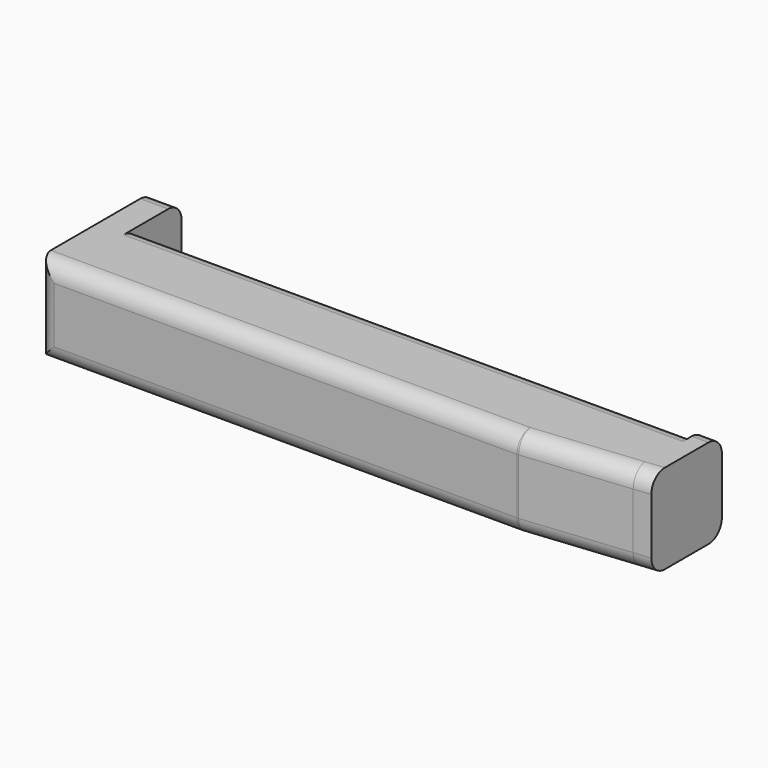
from build123d import *

# Parameters (mm, degrees)
F2_DEPTH      = 8
F2_DEPTH_BACK = 8
F3_R          = 3


# Not quite as in the source:
# - two fillets or chamfers of one size are made in one step


with BuildPart() as f2:
    # F1 (on Top) → F2 (new body, two sides)
    with BuildSketch(Plane.XY) as f2_sk:
        Polygon((-55, -8), (-50, -8), (-50, 8), (-50, 18), (-55, 18), align=None)
        Polygon((-50, -8), (30.9022613208, -8), (50, -6.0806050441), (50, 8), (-50, 8), align=None)
        Polygon((50, 8), (50, -6.0806050441), (53, -5.7790936996), (53, 10), (50, 10), align=None)
    extrude(amount=F2_DEPTH)
    extrude(f2_sk.sketch, amount=-F2_DEPTH_BACK)

    # F3 (call 1 of 7: OpenCascade refuses the feature's edges together)
    f3_edges = [f2.edges().sort_by_distance(p)[0] for p in [
        (-12.048869, -8, 8),
        (-55, -8, 0),
        (30.902261, -8, 0),
        (-12.048869, -8, -8),
        (41.951131, -6.889547, 8),
        (41.951131, -6.889547, -8),
    ]]
    fillet(f3_edges, radius=F3_R)

    # F3#2 (call 2 of 7)
    f3_2_edges = [f2.edges().sort_by_distance(p)[0] for p in [
        (-52.5, 18, -8),
    ]]
    fillet(f3_2_edges, radius=F3_R)

    # F3#3 (call 3 of 7)
    f3_3_edges = [f2.edges().sort_by_distance(p)[0] for p in [
        (-52.5, 18, 8),
    ]]
    fillet(f3_3_edges, radius=F3_R)

    # F3#4 (call 4 of 7)
    f3_4_edges = [f2.edges().sort_by_distance(p)[0] for p in [
        (0, 8, 8),
    ]]
    fillet(f3_4_edges, radius=F3_R)

    # F3#5 (call 5 of 7)
    f3_5_edges = [f2.edges().sort_by_distance(p)[0] for p in [
        (0, 8, -8),
    ]]
    fillet(f3_5_edges, radius=F3_R)

    # F3#6 (call 6 of 7)
    f3_6_edges = [f2.edges().sort_by_distance(p)[0] for p in [
        (51.5, 10, -8),
    ]]
    fillet(f3_6_edges, radius=F3_R)

    # F3#7 (call 7 of 7)
    f3_7_edges = [f2.edges().sort_by_distance(p)[0] for p in [
        (51.5, 10, 8),
    ]]
    fillet(f3_7_edges, radius=F3_R)


solid = f2.part
